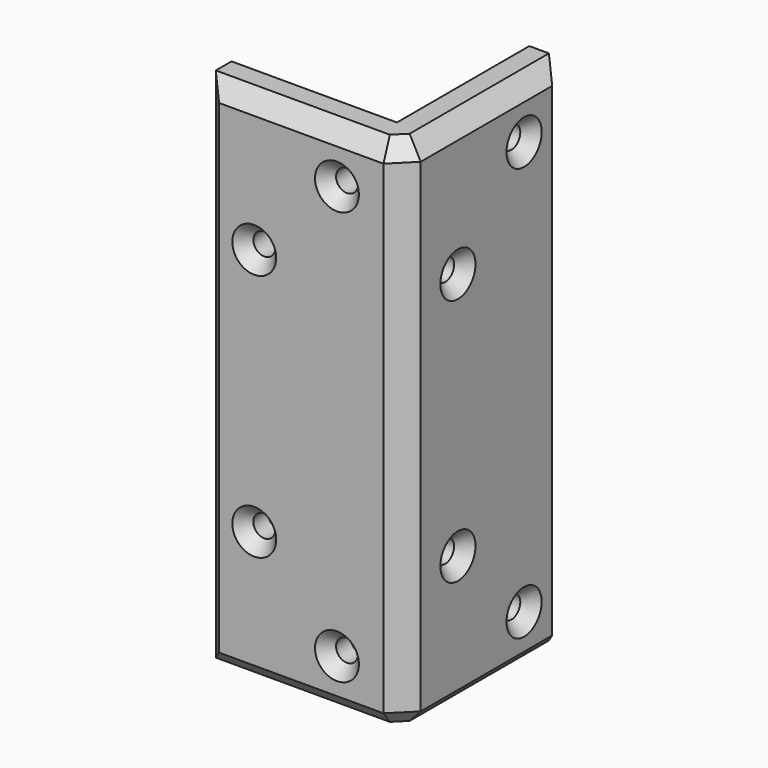
from build123d import *

# Parameters (mm, degrees)
F1_DEPTH             = 50.8
F2_W                 = 61.9125
F2_H                 = 61.9125
F3_DEPTH             = 57.15
F5_DEPTH             = 50.8
F8_D                 = 6.7564
F8_CSINK_D           = 13.4874
F8_CSINK_ANGLE       = 82
F8_ON_F7_D           = 6.7564
F8_ON_F7_CSINK_D     = 13.4874
F8_ON_F7_CSINK_ANGLE = 82
F9_SIZE              = 6.35
F11_SIZE             = 5.08


# Not quite as in the source:
# - a feature of the source that left no trace in its solid (it failed there, or was rolled back) is left out
# - a feature names something its author has since deleted; it is built from what else it names


with BuildPart() as f1:
    # F0 (on Top) → F1 (new body)
    with BuildSketch(Plane.XY):
        Polygon((-61.9125, 0), (0, 0), (0, 61.9125), (-11.1125, 61.9125), (-11.1125, 11.1125), (-61.9125, 11.1125), align=None)
    extrude(amount=F1_DEPTH)

    # F2 (on Top) → F3 (join)
    with BuildSketch(Plane.XY):
        with Locations((-30.95625, 30.95625)):
            Rectangle(F2_W, F2_H)
    extrude(amount=-F3_DEPTH)

    # F4 (on face) → F5 (join)
    with BuildSketch(Plane(origin=(0, 0, -57.15), x_dir=(1, 0, 0), z_dir=(0, 0, -1))):
        Polygon((0, -61.9125), (0, 0), (-61.9125, 0), (-61.9125, -9.525), (-9.525, -9.525), (-9.525, -61.9125), align=None)
    extrude(amount=F5_DEPTH)

    # F8 (through all)
    with Locations(Plane.YZ):
        with Locations((46.0375, 34.925), (20.6375, 9.525), (20.6375, -66.675), (46.0375, -92.075)):
            CounterSinkHole(F8_D / 2, F8_CSINK_D / 2, counter_sink_angle=F8_CSINK_ANGLE)

    # F8 on F7 (through all)
    with Locations(Plane.XZ):
        with Locations((-20.6375, 34.925), (-46.0375, 9.525), (-46.0375, -66.675), (-20.6375, -92.075)):
            CounterSinkHole(F8_ON_F7_D / 2, F8_ON_F7_CSINK_D / 2, counter_sink_angle=F8_ON_F7_CSINK_ANGLE)

    # F9
    f9_edges = [f1.edges().sort_by_distance(p)[0] for p in [
        (0, 0, -28.575),
    ]]
    chamfer(f9_edges, length=F9_SIZE)

    # F11
    f11_edges = [f1.edges().sort_by_distance(p)[0] for p in [
        (-34.13125, 0, 50.8),
        (-3.175, 3.175, 50.8),
        (0, 34.13125, 50.8),
        (-3.175, 3.175, -107.95),
        (-34.13125, 0, -107.95),
        (0, 34.13125, -107.95),
        (-61.9125, 0, -28.575),
        (0, 61.9125, -28.575),
    ]]
    chamfer(f11_edges, length=F11_SIZE)


solid = f1.part
